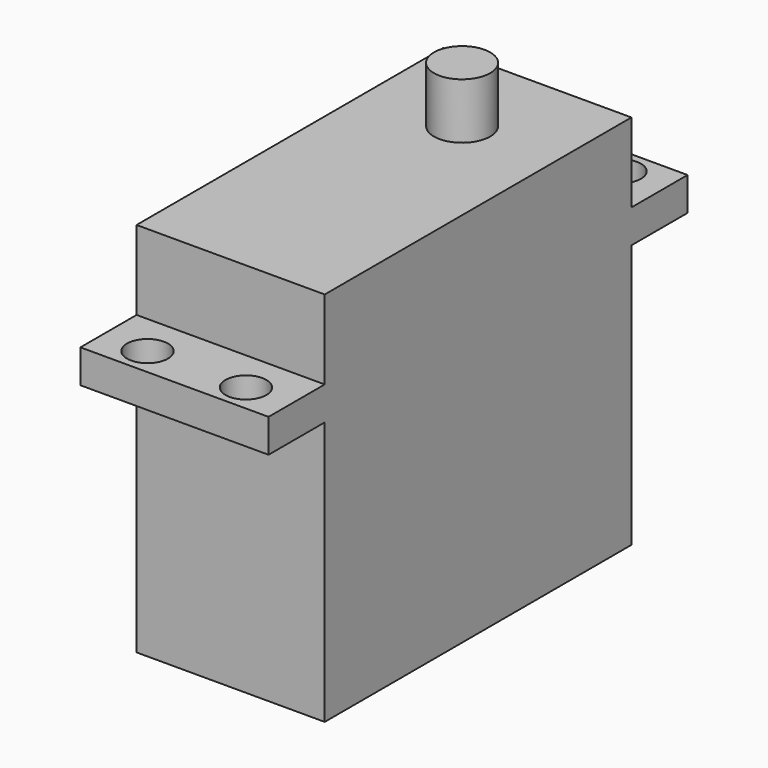
from build123d import *

# Parameters (mm, degrees)
F4_R          = 2.9337
F5_DEPTH      = 14.0716
F4_W          = 19.6088
F4_H          = 39.9542
F6_DEPTH      = 8.255
F6_DEPTH_BACK = 30.9626
F4_H_2        = 7.3152
F4_R_2        = 2.1336
F7_DEPTH      = 3.4798
F9_W          = 6.6548
F9_H          = 4.318
F10_DEPTH     = 7.62


# Not quite as in the source:
# - a variable given as a bare number and used for a length is read in inches; the dataset says mm whatever the document's units were


with BuildPart() as f5:
    # F4 (on Top) → F5 (new body)
    with BuildSketch(Plane.XY):
        with Locations((0, 10.1727)):
            Circle(F4_R)
    extrude(amount=F5_DEPTH)

    # F4 (on Top) → F6 (join, two sides)
    with BuildSketch(Plane.XY) as f6_sk:
        Rectangle(F4_W, F4_H)
        with Locations((0, 10.1727)):
            Circle(F4_R, mode=Mode.SUBTRACT)
        with Locations((0, 10.1727)):
            Circle(F4_R)
    extrude(amount=F6_DEPTH)
    extrude(f6_sk.sketch, amount=-F6_DEPTH_BACK)

    # F4 (on Top) → F7 (join)
    with BuildSketch(Plane.XY):
        with Locations((0, 23.6347)):
            Rectangle(F4_W, F4_H_2)
        with Locations((-5.1308, 24.3967)):
            Circle(F4_R_2, mode=Mode.SUBTRACT)
        with Locations((5.1308, 24.3967)):
            Circle(F4_R_2, mode=Mode.SUBTRACT)
        with Locations((0, -23.6347)):
            Rectangle(F4_W, F4_H_2)
        with Locations((-5.1308, -24.3967)):
            Circle(F4_R_2, mode=Mode.SUBTRACT)
        with Locations((5.1308, -24.3967)):
            Circle(F4_R_2, mode=Mode.SUBTRACT)
    extrude(amount=-F7_DEPTH)

    # F9 (on face) → F10 (join)
    with BuildSketch(Plane(origin=(0, 19.9771, 0), x_dir=(-1, 0, 0), z_dir=(0, 1, 0))):
        with Locations((0, -25.5016)):
            Rectangle(F9_W, F9_H)
    extrude(amount=F10_DEPTH)


solid = f5.part
